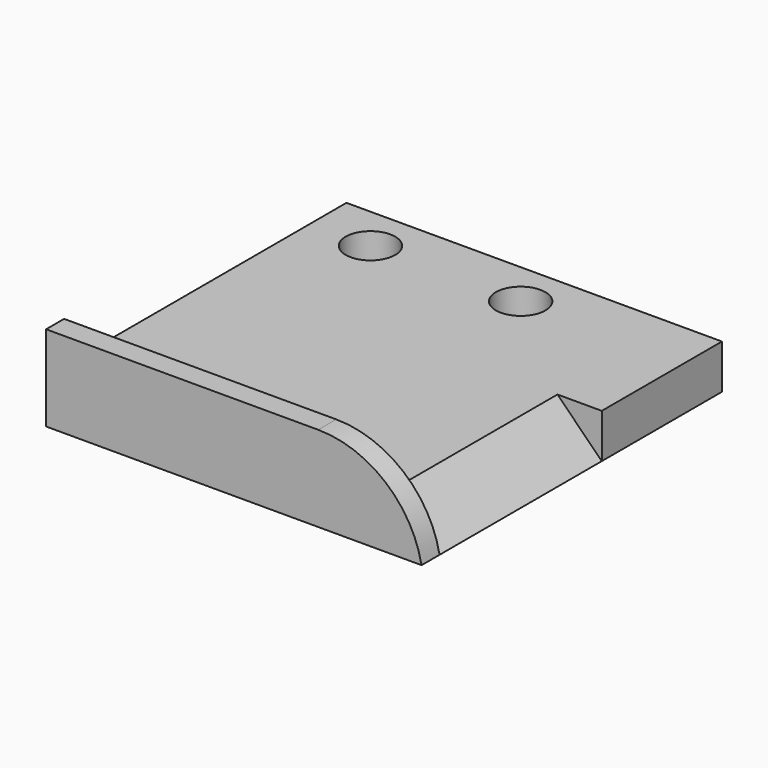
from build123d import *

# Parameters (mm, degrees)
F0_W        = 12.5
F0_H        = 25
F1_DEPTH    = 5.7
F2_W        = 23.5
F2_H        = 2.75
F3_DEPTH    = 25.001
F5_DEPTH    = 13.5
F6_T1_DEPTH = 18.695566289
F7_R        = 1.65
F8_DEPTH    = 25


# Not quite as in the source:
# - a fillet or chamfer that OpenCascade refuses, or shapes differently, is made with other operations: its cross-section is extruded or revolved along the edge and cut away or added


with BuildPart() as f1:
    # F0 (on Top) → F1 (new body)
    with BuildSketch(Plane.XY):
        with Locations((-6.25, 12.5)):
            Rectangle(F0_W, F0_H)
        with Locations((6.25, 12.5)):
            Rectangle(F0_W, F0_H)
    extrude(amount=F1_DEPTH)

    # F2 (on face) → F3 (cut, through all)
    with BuildSketch(Plane(origin=(-12.5, 0, 0), x_dir=(0, -1, 0), z_dir=(-1, 0, 0))):
        with Locations((-13.25, 4.325)):
            Rectangle(F2_W, F2_H)
    extrude(amount=-F3_DEPTH, mode=Mode.SUBTRACT)

    # F4 (on face) → F5 (cut)
    with BuildSketch(Plane(origin=(0, 1.5, 0), x_dir=(-1, 0, 0), z_dir=(0, 1, 0))):
        Polygon((-9.55, 2.95), (-12.5, 2.95), (-12.5, 0), align=None)
    extrude(amount=F5_DEPTH, mode=Mode.SUBTRACT)

    # F6: fillet of radius 7 on 1 edges, made by hand

    # F6_s2 → F6_t1 (cut)
    with BuildSketch(Plane.XZ.offset(-1.5)):
        with BuildLine():
            ThreePointArc((12.5, 0), (10.0883157712, 4.0898051913), (5.6217734844, 5.7))
            Line((5.6217734844, 5.7), (12.5, 5.7))
            Line((12.5, 5.7), (12.5, 0))
        make_face()
    extrude(amount=F6_T1_DEPTH, mode=Mode.SUBTRACT)

    # F7 (on face) → F8 (cut)
    with BuildSketch(Plane.XY.offset(2.95)):
        with Locations((-8.5, 22)):
            Circle(F7_R)
        with Locations((1.5, 22)):
            Circle(F7_R)
    extrude(amount=-F8_DEPTH, mode=Mode.SUBTRACT)


solid = f1.part
